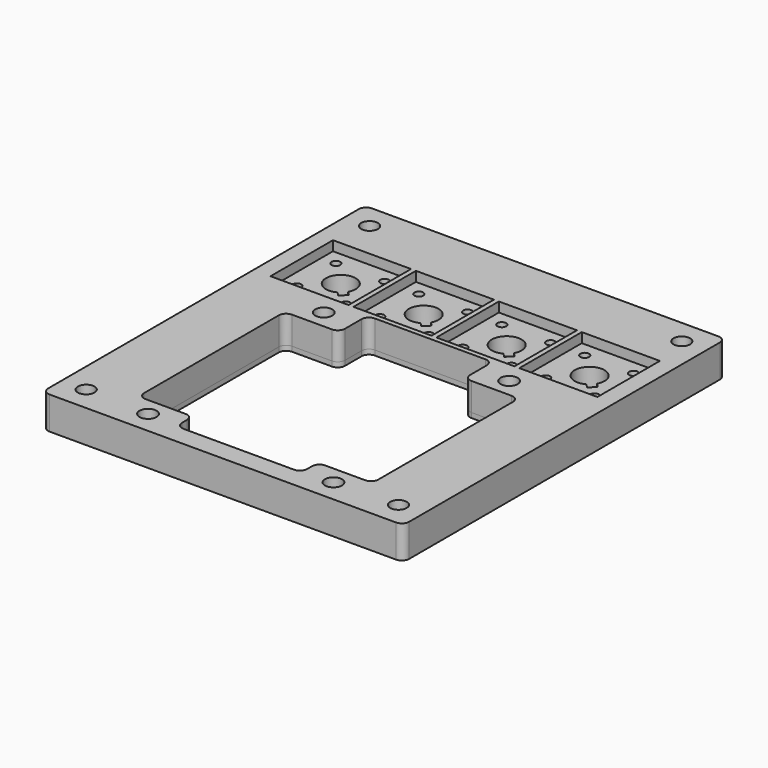
from build123d import *

# Parameters (mm, degrees)
F1_R     = 3
F1_R_2   = 1.75
F1_R_3   = 0.9
F1_R_4   = 1.7
F2_DEPTH = 5.7
F1_R_5   = 0.4
F3_DEPTH = 1
F4_W     = 16
F4_H     = 16
F5_DEPTH = 2
F6_R     = 1.5


with BuildPart() as f2:
    # F1 (on Top) → F2 (new body)
    with BuildSketch(Plane.XY):
        Polygon((-37, 10.5), (-37, -62.1), (37, -62.1), (37, 10.5), (37, 20.5), (-37, 20.5), align=None)
        with Locations((-32, -57.1)):
            Circle(F1_R, mode=Mode.SUBTRACT)
        with Locations((-19, -57.5)):
            Circle(F1_R_2, mode=Mode.SUBTRACT)
        with Locations((19, -57.5)):
            Circle(F1_R_2, mode=Mode.SUBTRACT)
        with Locations((32, -57.1)):
            Circle(F1_R, mode=Mode.SUBTRACT)
        Polygon((-24, -53.75), (-24, -16.25), (-12.8245735195, -16.25), (-12.8245735195, -9), (12.8245735195, -9), (12.8245735195, -16.25), (24, -16.25), (24, -53.75), (12.8245735195, -53.75), (12.8245735195, -58), (-12.8245735195, -58), (-12.8245735195, -53.75), align=None, mode=Mode.SUBTRACT)
        with Locations((-19, -12.5)):
            Circle(F1_R_2, mode=Mode.SUBTRACT)
        with Locations((-30.5, -5)):
            Circle(F1_R_3, mode=Mode.SUBTRACT)
        with BuildLine():
            Line((-22.6362171983, -2.8637828017), (-23.2372583002, -3.4648239035))
            Line((-23.2372583002, -3.4648239035), (-24.0298093304, -2.6722728733))
            ThreePointArc((-24.0298093304, -2.6722728733), (-27.6566760205, 2.1566760205), (-22.8277271267, -1.4701906696))
            Line((-22.8277271267, -1.4701906696), (-22.0351760965, -2.2627416998))
            Line((-22.0351760965, -2.2627416998), (-22.6362171983, -2.8637828017))
        make_face(mode=Mode.SUBTRACT)
        with Locations((-20.5, -5)):
            Circle(F1_R_3, mode=Mode.SUBTRACT)
        with Locations((-13.5, -5)):
            Circle(F1_R_3, mode=Mode.SUBTRACT)
        with BuildLine():
            ThreePointArc((-7.0298093304, -2.6722728733), (-10.6566760205, 2.1566760205), (-5.8277271267, -1.4701906696))
            Line((-5.8277271267, -1.4701906696), (-5.0351760965, -2.2627416998))
            Line((-5.0351760965, -2.2627416998), (-5.6362171983, -2.8637828017))
            Line((-5.6362171983, -2.8637828017), (-6.2372583002, -3.4648239035))
            Line((-6.2372583002, -3.4648239035), (-7.0298093304, -2.6722728733))
        make_face(mode=Mode.SUBTRACT)
        with Locations((-3.5, -5)):
            Circle(F1_R_3, mode=Mode.SUBTRACT)
        with Locations((-30.5, 5)):
            Circle(F1_R_3, mode=Mode.SUBTRACT)
        with Locations((-20.5, 5)):
            Circle(F1_R_3, mode=Mode.SUBTRACT)
        with Locations((-32, 15.5)):
            Circle(F1_R, mode=Mode.SUBTRACT)
        with Locations((-13.5, 5)):
            Circle(F1_R_3, mode=Mode.SUBTRACT)
        with Locations((-3.5, 5)):
            Circle(F1_R_3, mode=Mode.SUBTRACT)
        with Locations((3.5, -5)):
            Circle(F1_R_3, mode=Mode.SUBTRACT)
        with BuildLine():
            ThreePointArc((9.9701906696, -2.6722728733), (6.3433239795, 2.1566760205), (11.1722728733, -1.4701906696))
            Line((11.1722728733, -1.4701906696), (11.9648239035, -2.2627416998))
            Line((11.9648239035, -2.2627416998), (11.3637828017, -2.8637828017))
            Line((11.3637828017, -2.8637828017), (10.7627416998, -3.4648239035))
            Line((10.7627416998, -3.4648239035), (9.9701906696, -2.6722728733))
        make_face(mode=Mode.SUBTRACT)
        with Locations((13.5, -5)):
            Circle(F1_R_3, mode=Mode.SUBTRACT)
        with Locations((19, -12.5)):
            Circle(F1_R_2, mode=Mode.SUBTRACT)
        with Locations((20.5, -5)):
            Circle(F1_R_3, mode=Mode.SUBTRACT)
        with BuildLine():
            ThreePointArc((26.9701906696, -2.6722728733), (23.3433239795, 2.1566760205), (28.1722728733, -1.4701906696))
            Line((28.1722728733, -1.4701906696), (28.9648239035, -2.2627416998))
            Line((28.9648239035, -2.2627416998), (28.3637828017, -2.8637828017))
            Line((28.3637828017, -2.8637828017), (27.7627416998, -3.4648239035))
            Line((27.7627416998, -3.4648239035), (26.9701906696, -2.6722728733))
        make_face(mode=Mode.SUBTRACT)
        with Locations((30.5, -5)):
            Circle(F1_R_3, mode=Mode.SUBTRACT)
        with Locations((3.5, 5)):
            Circle(F1_R_3, mode=Mode.SUBTRACT)
        with Locations((13.5, 5)):
            Circle(F1_R_3, mode=Mode.SUBTRACT)
        with Locations((20.5, 5)):
            Circle(F1_R_3, mode=Mode.SUBTRACT)
        with Locations((30.5, 5)):
            Circle(F1_R_3, mode=Mode.SUBTRACT)
        with Locations((32, 15.5)):
            Circle(F1_R, mode=Mode.SUBTRACT)
        with Locations((-32, 15.5)):
            Circle(F1_R)
        with Locations((-32, 15.5)):
            Circle(F1_R_4, mode=Mode.SUBTRACT)
        with Locations((32, 15.5)):
            Circle(F1_R)
        with Locations((32, 15.5)):
            Circle(F1_R_4, mode=Mode.SUBTRACT)
        with Locations((-32, -57.1)):
            Circle(F1_R)
        with Locations((-32, -57.1)):
            Circle(F1_R_4, mode=Mode.SUBTRACT)
        with Locations((32, -57.1)):
            Circle(F1_R)
        with Locations((32, -57.1)):
            Circle(F1_R_4, mode=Mode.SUBTRACT)
    extrude(amount=F2_DEPTH)

    # F1 (on Top) → F3 (join)
    with BuildSketch(Plane.XY):
        Polygon((-37, 10.5), (-37, -62.1), (37, -62.1), (37, 10.5), (37, 20.5), (-37, 20.5), align=None)
        with Locations((-32, -57.1)):
            Circle(F1_R, mode=Mode.SUBTRACT)
        with Locations((-19, -57.5)):
            Circle(F1_R_2, mode=Mode.SUBTRACT)
        with Locations((19, -57.5)):
            Circle(F1_R_2, mode=Mode.SUBTRACT)
        with Locations((32, -57.1)):
            Circle(F1_R, mode=Mode.SUBTRACT)
        Polygon((-24, -53.75), (-24, -16.25), (-12.8245735195, -16.25), (-12.8245735195, -9), (12.8245735195, -9), (12.8245735195, -16.25), (24, -16.25), (24, -53.75), (12.8245735195, -53.75), (12.8245735195, -58), (-12.8245735195, -58), (-12.8245735195, -53.75), align=None, mode=Mode.SUBTRACT)
        with Locations((-19, -12.5)):
            Circle(F1_R_2, mode=Mode.SUBTRACT)
        with Locations((-30.5, -5)):
            Circle(F1_R_3, mode=Mode.SUBTRACT)
        with BuildLine():
            Line((-22.6362171983, -2.8637828017), (-23.2372583002, -3.4648239035))
            Line((-23.2372583002, -3.4648239035), (-24.0298093304, -2.6722728733))
            ThreePointArc((-24.0298093304, -2.6722728733), (-27.6566760205, 2.1566760205), (-22.8277271267, -1.4701906696))
            Line((-22.8277271267, -1.4701906696), (-22.0351760965, -2.2627416998))
            Line((-22.0351760965, -2.2627416998), (-22.6362171983, -2.8637828017))
        make_face(mode=Mode.SUBTRACT)
        with Locations((-20.5, -5)):
            Circle(F1_R_3, mode=Mode.SUBTRACT)
        with Locations((-13.5, -5)):
            Circle(F1_R_3, mode=Mode.SUBTRACT)
        with BuildLine():
            ThreePointArc((-7.0298093304, -2.6722728733), (-10.6566760205, 2.1566760205), (-5.8277271267, -1.4701906696))
            Line((-5.8277271267, -1.4701906696), (-5.0351760965, -2.2627416998))
            Line((-5.0351760965, -2.2627416998), (-5.6362171983, -2.8637828017))
            Line((-5.6362171983, -2.8637828017), (-6.2372583002, -3.4648239035))
            Line((-6.2372583002, -3.4648239035), (-7.0298093304, -2.6722728733))
        make_face(mode=Mode.SUBTRACT)
        with Locations((-3.5, -5)):
            Circle(F1_R_3, mode=Mode.SUBTRACT)
        with Locations((-30.5, 5)):
            Circle(F1_R_3, mode=Mode.SUBTRACT)
        with Locations((-20.5, 5)):
            Circle(F1_R_3, mode=Mode.SUBTRACT)
        with Locations((-32, 15.5)):
            Circle(F1_R, mode=Mode.SUBTRACT)
        with Locations((-13.5, 5)):
            Circle(F1_R_3, mode=Mode.SUBTRACT)
        with Locations((-3.5, 5)):
            Circle(F1_R_3, mode=Mode.SUBTRACT)
        with Locations((3.5, -5)):
            Circle(F1_R_3, mode=Mode.SUBTRACT)
        with BuildLine():
            ThreePointArc((9.9701906696, -2.6722728733), (6.3433239795, 2.1566760205), (11.1722728733, -1.4701906696))
            Line((11.1722728733, -1.4701906696), (11.9648239035, -2.2627416998))
            Line((11.9648239035, -2.2627416998), (11.3637828017, -2.8637828017))
            Line((11.3637828017, -2.8637828017), (10.7627416998, -3.4648239035))
            Line((10.7627416998, -3.4648239035), (9.9701906696, -2.6722728733))
        make_face(mode=Mode.SUBTRACT)
        with Locations((13.5, -5)):
            Circle(F1_R_3, mode=Mode.SUBTRACT)
        with Locations((19, -12.5)):
            Circle(F1_R_2, mode=Mode.SUBTRACT)
        with Locations((20.5, -5)):
            Circle(F1_R_3, mode=Mode.SUBTRACT)
        with BuildLine():
            ThreePointArc((26.9701906696, -2.6722728733), (23.3433239795, 2.1566760205), (28.1722728733, -1.4701906696))
            Line((28.1722728733, -1.4701906696), (28.9648239035, -2.2627416998))
            Line((28.9648239035, -2.2627416998), (28.3637828017, -2.8637828017))
            Line((28.3637828017, -2.8637828017), (27.7627416998, -3.4648239035))
            Line((27.7627416998, -3.4648239035), (26.9701906696, -2.6722728733))
        make_face(mode=Mode.SUBTRACT)
        with Locations((30.5, -5)):
            Circle(F1_R_3, mode=Mode.SUBTRACT)
        with Locations((3.5, 5)):
            Circle(F1_R_3, mode=Mode.SUBTRACT)
        with Locations((13.5, 5)):
            Circle(F1_R_3, mode=Mode.SUBTRACT)
        with Locations((20.5, 5)):
            Circle(F1_R_3, mode=Mode.SUBTRACT)
        with Locations((30.5, 5)):
            Circle(F1_R_3, mode=Mode.SUBTRACT)
        with Locations((32, 15.5)):
            Circle(F1_R, mode=Mode.SUBTRACT)
        with BuildLine():
            Line((-24.0298093304, -2.6722728733), (-23.2372583002, -3.4648239035))
            Line((-23.2372583002, -3.4648239035), (-22.6362171983, -2.8637828017))
            Line((-22.6362171983, -2.8637828017), (-22.0351760965, -2.2627416998))
            Line((-22.0351760965, -2.2627416998), (-22.8277271267, -1.4701906696))
            ThreePointArc((-22.8277271267, -1.4701906696), (-27.6566760205, 2.1566760205), (-24.0298093304, -2.6722728733))
        make_face()
        with Locations((-26.77, 0)):
            Circle(F1_R_5, mode=Mode.SUBTRACT)
        with Locations((-25.5, 1.27)):
            Circle(F1_R_5, mode=Mode.SUBTRACT)
        with Locations((-24.23, 0)):
            Circle(F1_R_5, mode=Mode.SUBTRACT)
        with BuildLine():
            Line((-5.0351760965, -2.2627416998), (-5.8277271267, -1.4701906696))
            ThreePointArc((-5.8277271267, -1.4701906696), (-10.6566760205, 2.1566760205), (-7.0298093304, -2.6722728733))
            Line((-7.0298093304, -2.6722728733), (-6.2372583002, -3.4648239035))
            Line((-6.2372583002, -3.4648239035), (-5.6362171983, -2.8637828017))
            Line((-5.6362171983, -2.8637828017), (-5.0351760965, -2.2627416998))
        make_face()
        with Locations((-9.77, 0)):
            Circle(F1_R_5, mode=Mode.SUBTRACT)
        with Locations((-7.23, 0)):
            Circle(F1_R_5, mode=Mode.SUBTRACT)
        with Locations((-8.5, 1.27)):
            Circle(F1_R_5, mode=Mode.SUBTRACT)
        with BuildLine():
            Line((11.9648239035, -2.2627416998), (11.1722728733, -1.4701906696))
            ThreePointArc((11.1722728733, -1.4701906696), (6.3433239795, 2.1566760205), (9.9701906696, -2.6722728733))
            Line((9.9701906696, -2.6722728733), (10.7627416998, -3.4648239035))
            Line((10.7627416998, -3.4648239035), (11.3637828017, -2.8637828017))
            Line((11.3637828017, -2.8637828017), (11.9648239035, -2.2627416998))
        make_face()
        with Locations((7.23, 0)):
            Circle(F1_R_5, mode=Mode.SUBTRACT)
        with Locations((8.5, 1.27)):
            Circle(F1_R_5, mode=Mode.SUBTRACT)
        with Locations((9.77, 0)):
            Circle(F1_R_5, mode=Mode.SUBTRACT)
        with BuildLine():
            Line((28.9648239035, -2.2627416998), (28.1722728733, -1.4701906696))
            ThreePointArc((28.1722728733, -1.4701906696), (23.3433239795, 2.1566760205), (26.9701906696, -2.6722728733))
            Line((26.9701906696, -2.6722728733), (27.7627416998, -3.4648239035))
            Line((27.7627416998, -3.4648239035), (28.3637828017, -2.8637828017))
            Line((28.3637828017, -2.8637828017), (28.9648239035, -2.2627416998))
        make_face()
        with Locations((24.23, 0)):
            Circle(F1_R_5, mode=Mode.SUBTRACT)
        with Locations((26.77, 0)):
            Circle(F1_R_5, mode=Mode.SUBTRACT)
        with Locations((25.5, 1.27)):
            Circle(F1_R_5, mode=Mode.SUBTRACT)
        with Locations((-32, -57.1)):
            Circle(F1_R)
        with Locations((-32, -57.1)):
            Circle(F1_R_4, mode=Mode.SUBTRACT)
        with Locations((-32, 15.5)):
            Circle(F1_R)
        with Locations((-32, 15.5)):
            Circle(F1_R_4, mode=Mode.SUBTRACT)
        with Locations((32, 15.5)):
            Circle(F1_R)
        with Locations((32, 15.5)):
            Circle(F1_R_4, mode=Mode.SUBTRACT)
        with Locations((32, -57.1)):
            Circle(F1_R)
        with Locations((32, -57.1)):
            Circle(F1_R_4, mode=Mode.SUBTRACT)
    extrude(amount=-F3_DEPTH)

    # F4 (on face) → F5 (cut)
    with BuildSketch(Plane.XY.offset(5.7)):
        with Locations((-25.5, 0)):
            Rectangle(F4_W, F4_H)
        with Locations((-8.5, 0)):
            Rectangle(F4_W, F4_H)
        with Locations((8.5, 0)):
            Rectangle(F4_W, F4_H)
        with Locations((25.5, 0)):
            Rectangle(F4_W, F4_H)
    extrude(amount=-F5_DEPTH, mode=Mode.SUBTRACT)

    # F6
    f6_edges = [f2.edges().sort_by_distance(p)[0] for p in [
        (-12.824574, -16.25, 2.35),
        (12.824574, -16.25, 2.35),
        (-12.824574, -9, 2.35),
        (12.824574, -9, 2.35),
        (24, -16.25, 2.35),
        (-24, -16.25, 2.35),
        (-24, -53.75, 2.35),
        (-12.824574, -53.75, 2.35),
        (-12.824574, -58, 2.35),
        (12.824574, -58, 2.35),
        (12.824574, -53.75, 2.35),
        (24, -53.75, 2.35),
        (-37, -62.1, 2.35),
        (37, -62.1, 2.35),
        (-37, 20.5, 2.35),
        (37, 20.5, 2.35),
    ]]
    fillet(f6_edges, radius=F6_R)


solid = f2.part
